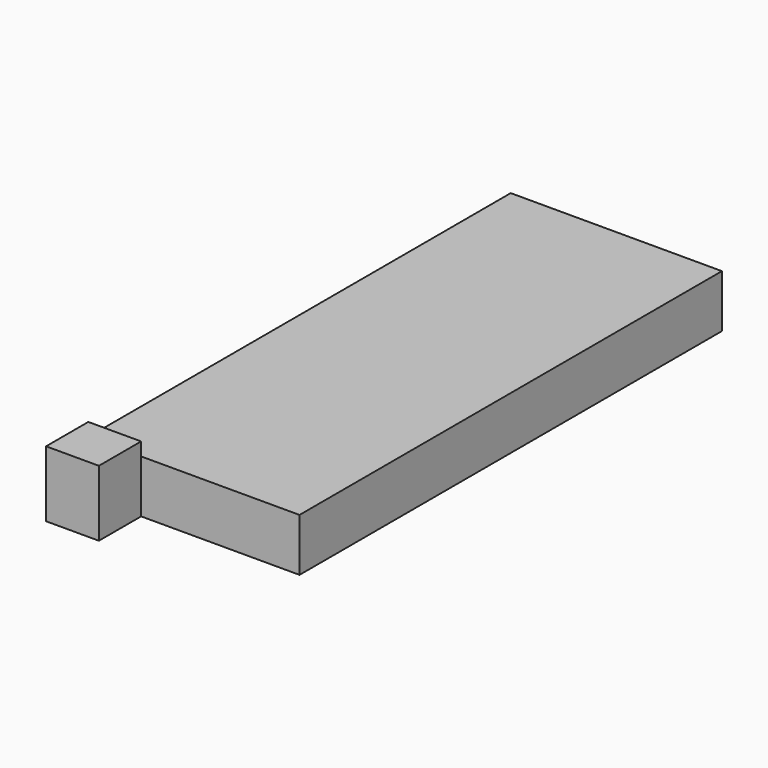
from build123d import *

# Parameters (mm, degrees)
F0_W     = 20
F0_H     = 20
F1_DEPTH = 20
F2_DEPTH = 200
F3_DEPTH = 5
F4_DEPTH = 20
F5_DEPTH = 40


with BuildPart() as f1:
    # F0 (on Top) → F1 (new body)
    with BuildSketch(Plane.XY):
        with Locations((10, 10)):
            Rectangle(F0_W, F0_H)
    extrude(amount=F1_DEPTH)


with BuildPart() as f2:
    # F2 (new): a face of the model
    f2_faces = [f1.part.faces().sort_by_distance(p)[0] for p in [
        (10, 20, 10),
    ]]
    extrude(f2_faces, amount=F2_DEPTH)

    # F4 (add): a face of the model
    f4_faces = [f2.faces().sort_by_distance(p)[0] for p in [
        (20, 120, 10),
    ]]
    extrude(f4_faces, amount=F4_DEPTH)

    # F5 (add): a face of the model
    f5_faces = [f2.faces().sort_by_distance(p)[0] for p in [
        (40, 120, 10),
    ]]
    extrude(f5_faces, amount=F5_DEPTH)


with BuildPart() as f1_1:
    add(f1.part)

    # F3 (add): a face of the model
    f3_faces = [f1_1.faces().sort_by_distance(p)[0] for p in [
        (10, 10, 20),
    ]]
    extrude(f3_faces, amount=F3_DEPTH)


solid = Compound([f2.part, f1_1.part])
